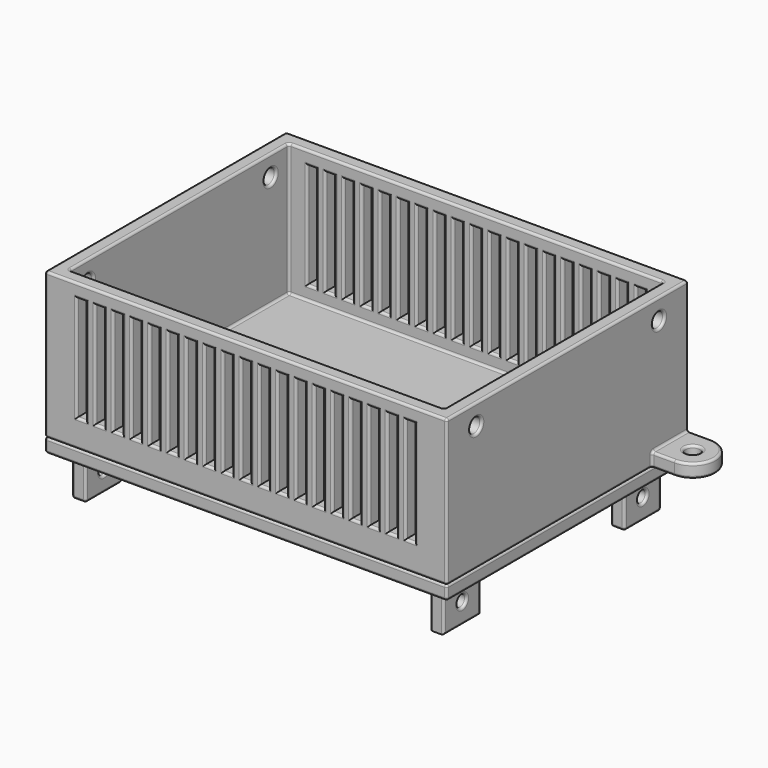
from build123d import *

# Parameters (mm, degrees)
F5_W           = 82
F5_H           = 60
F6_DEPTH       = 32
F5_W_2         = 3
F5_H_2         = 10
F5_W_3         = 2
F5_H_3         = 3
F5_R           = 3.5
F5_R_2         = 1.6
F7_DEPTH       = 3
F8_DEPTH       = 3
F9_DEPTH       = 1
F10_DEPTH      = 12
F11_DEPTH      = 1
F12_R          = 1.25
F12_R_2        = 1.6
F13_DEPTH      = 85
F13_DEPTH_BACK = 3
F14_W          = 2
F14_H          = 23
F15_DEPTH      = 3
F15_DEPTH_BACK = 63
F16_R          = 0.5
F16_2_R        = 0.5


with BuildPart() as f6:
    # F5 (on Top) → F6 (new body)
    with BuildSketch(Plane.XY):
        Polygon((85, 3), (-3, 3), (-3, -7), (-3, -63), (85, -63), (85, -7), align=None)
        with Locations((41, -30)):
            Rectangle(F5_W, F5_H, mode=Mode.SUBTRACT)
    extrude(amount=F6_DEPTH)

    # F5 (on Top) → F7 (join)
    with BuildSketch(Plane.XY):
        with Locations((41, -30)):
            Rectangle(F5_W, F5_H)
        with Locations((1.8, -54.7)):
            Rectangle(F5_W_2, F5_H_2, mode=Mode.SUBTRACT)
        Polygon((5.4330127019, -46.6423048454), (5, -46.3923048454), (4.5669872981, -46.1423048454), (6.0669872981, -43.5442286341), (6.9330127019, -44.0442286341), align=None, mode=Mode.SUBTRACT)
        with Locations((3, -36)):
            Rectangle(F5_W_3, F5_H_3, mode=Mode.SUBTRACT)
        with Locations((11, -36)):
            Circle(F5_R, mode=Mode.SUBTRACT)
        Polygon((17, -46.3923048454), (16.5669872981, -46.6423048454), (15.0669872981, -44.0442286341), (15.9330127019, -43.5442286341), (17.4330127019, -46.1423048454), align=None, mode=Mode.SUBTRACT)
        Polygon((26.0669872981, -43.5442286341), (26.9330127019, -44.0442286341), (25.4330127019, -46.6423048454), (25, -46.3923048454), (24.5669872981, -46.1423048454), align=None, mode=Mode.SUBTRACT)
        Polygon((35.9330127019, -43.5442286341), (37.4330127019, -46.1423048454), (37, -46.3923048454), (36.5669872981, -46.6423048454), (35.0669872981, -44.0442286341), align=None, mode=Mode.SUBTRACT)
        with Locations((19, -36)):
            Rectangle(F5_W_3, F5_H_3, mode=Mode.SUBTRACT)
        with Locations((23, -36)):
            Rectangle(F5_W_3, F5_H_3, mode=Mode.SUBTRACT)
        with Locations((31, -36)):
            Circle(F5_R, mode=Mode.SUBTRACT)
        with Locations((39, -36)):
            Rectangle(F5_W_3, F5_H_3, mode=Mode.SUBTRACT)
        with Locations((80.2, -54.7)):
            Rectangle(F5_W_2, F5_H_2, mode=Mode.SUBTRACT)
        Polygon((46.0669872981, -43.5442286341), (46.9330127019, -44.0442286341), (45.4330127019, -46.6423048454), (45, -46.3923048454), (44.5669872981, -46.1423048454), align=None, mode=Mode.SUBTRACT)
        Polygon((55.9330127019, -43.5442286341), (57.4330127019, -46.1423048454), (57, -46.3923048454), (56.5669872981, -46.6423048454), (55.0669872981, -44.0442286341), align=None, mode=Mode.SUBTRACT)
        Polygon((66.0669872981, -43.5442286341), (66.9330127019, -44.0442286341), (65.4330127019, -46.6423048454), (65, -46.3923048454), (64.5669872981, -46.1423048454), align=None, mode=Mode.SUBTRACT)
        with Locations((43, -36)):
            Rectangle(F5_W_3, F5_H_3, mode=Mode.SUBTRACT)
        with Locations((51, -36)):
            Circle(F5_R, mode=Mode.SUBTRACT)
        with Locations((59, -36)):
            Rectangle(F5_W_3, F5_H_3, mode=Mode.SUBTRACT)
        with Locations((63, -36)):
            Rectangle(F5_W_3, F5_H_3, mode=Mode.SUBTRACT)
        Polygon((75.9330127019, -43.5442286341), (77.4330127019, -46.1423048454), (77, -46.3923048454), (76.5669872981, -46.6423048454), (75.0669872981, -44.0442286341), align=None, mode=Mode.SUBTRACT)
        with Locations((71, -36)):
            Circle(F5_R, mode=Mode.SUBTRACT)
        with Locations((79, -36)):
            Rectangle(F5_W_3, F5_H_3, mode=Mode.SUBTRACT)
        Polygon((11.5, -27), (11, -27), (10.5, -27), (10.5, -24), (11.5, -24), align=None, mode=Mode.SUBTRACT)
        Polygon((31.5, -24), (31.5, -27), (31, -27), (30.5, -27), (30.5, -24), align=None, mode=Mode.SUBTRACT)
        with Locations((1.8, -5.3)):
            Rectangle(F5_W_2, F5_H_2, mode=Mode.SUBTRACT)
        Polygon((51.5, -24), (51.5, -27), (51, -27), (50.5, -27), (50.5, -24), align=None, mode=Mode.SUBTRACT)
        Polygon((71.5, -24), (71.5, -27), (71, -27), (70.5, -27), (70.5, -24), align=None, mode=Mode.SUBTRACT)
        with Locations((80.2, -5.3)):
            Rectangle(F5_W_2, F5_H_2, mode=Mode.SUBTRACT)
        with Locations((1.8, -5.3)):
            Rectangle(F5_W_2, F5_H_2)
        with Locations((1.8, -54.7)):
            Rectangle(F5_W_2, F5_H_2)
        with Locations((3, -36)):
            Rectangle(F5_W_3, F5_H_3)
        with Locations((11, -36)):
            Circle(F5_R)
        with Locations((19, -36)):
            Rectangle(F5_W_3, F5_H_3)
        with Locations((23, -36)):
            Rectangle(F5_W_3, F5_H_3)
        with Locations((31, -36)):
            Circle(F5_R)
        with Locations((39, -36)):
            Rectangle(F5_W_3, F5_H_3)
        with Locations((43, -36)):
            Rectangle(F5_W_3, F5_H_3)
        with Locations((51, -36)):
            Circle(F5_R)
        with Locations((63, -36)):
            Rectangle(F5_W_3, F5_H_3)
        with Locations((59, -36)):
            Rectangle(F5_W_3, F5_H_3)
        with Locations((71, -36)):
            Circle(F5_R)
        with Locations((79, -36)):
            Rectangle(F5_W_3, F5_H_3)
        with Locations((80.2, -5.3)):
            Rectangle(F5_W_2, F5_H_2)
        with Locations((80.2, -54.7)):
            Rectangle(F5_W_2, F5_H_2)
        Polygon((4.5669872981, -46.1423048454), (5, -46.3923048454), (5.4330127019, -46.6423048454), (6.9330127019, -44.0442286341), (6.0669872981, -43.5442286341), align=None)
        Polygon((15.0669872981, -44.0442286341), (16.5669872981, -46.6423048454), (17, -46.3923048454), (17.4330127019, -46.1423048454), (15.9330127019, -43.5442286341), align=None)
        Polygon((10.5, -27), (11, -27), (11.5, -27), (11.5, -24), (10.5, -24), align=None)
        Polygon((37, -46.3923048454), (37.4330127019, -46.1423048454), (35.9330127019, -43.5442286341), (35.0669872981, -44.0442286341), (36.5669872981, -46.6423048454), align=None)
        Polygon((51, -27), (51.5, -27), (51.5, -24), (50.5, -24), (50.5, -27), align=None)
        Polygon((45.4330127019, -46.6423048454), (46.9330127019, -44.0442286341), (46.0669872981, -43.5442286341), (44.5669872981, -46.1423048454), (45, -46.3923048454), align=None)
        Polygon((57, -46.3923048454), (57.4330127019, -46.1423048454), (55.9330127019, -43.5442286341), (55.0669872981, -44.0442286341), (56.5669872981, -46.6423048454), align=None)
        Polygon((71, -27), (71.5, -27), (71.5, -24), (70.5, -24), (70.5, -27), align=None)
        Polygon((65.4330127019, -46.6423048454), (66.9330127019, -44.0442286341), (66.0669872981, -43.5442286341), (64.5669872981, -46.1423048454), (65, -46.3923048454), align=None)
        Polygon((77, -46.3923048454), (77.4330127019, -46.1423048454), (75.9330127019, -43.5442286341), (75.0669872981, -44.0442286341), (76.5669872981, -46.6423048454), align=None)
        Polygon((31, -27), (31.5, -27), (31.5, -24), (30.5, -24), (30.5, -27), align=None)
        Polygon((25.4330127019, -46.6423048454), (26.9330127019, -44.0442286341), (26.0669872981, -43.5442286341), (24.5669872981, -46.1423048454), (25, -46.3923048454), align=None)
        with BuildLine():
            Line((-3, -7), (-3, 3))
            Line((-3, 3), (-8, 3))
            ThreePointArc((-8, 3), (-13, -2), (-8, -7))
            Line((-8, -7), (-3, -7))
        make_face()
        with Locations((-8, -2)):
            Circle(F5_R_2, mode=Mode.SUBTRACT)
        with BuildLine():
            Line((90, 3), (85, 3))
            Line((85, 3), (85, -7))
            Line((85, -7), (90, -7))
            ThreePointArc((90, -7), (95, -2), (90, 3))
        make_face()
        with Locations((90, -2)):
            Circle(F5_R_2, mode=Mode.SUBTRACT)
    extrude(amount=F7_DEPTH)


with BuildPart() as f8:
    # F5 (on Top) → F8 (new body)
    with BuildSketch(Plane.XY):
        Polygon((85, 3), (-3, 3), (-3, -7), (-3, -63), (85, -63), (85, -7), align=None)
        with Locations((41, -30)):
            Rectangle(F5_W, F5_H, mode=Mode.SUBTRACT)
        with Locations((41, -30)):
            Rectangle(F5_W, F5_H)
        with Locations((1.8, -54.7)):
            Rectangle(F5_W_2, F5_H_2, mode=Mode.SUBTRACT)
        Polygon((5.4330127019, -46.6423048454), (5, -46.3923048454), (4.5669872981, -46.1423048454), (6.0669872981, -43.5442286341), (6.9330127019, -44.0442286341), align=None, mode=Mode.SUBTRACT)
        with Locations((3, -36)):
            Rectangle(F5_W_3, F5_H_3, mode=Mode.SUBTRACT)
        with Locations((11, -36)):
            Circle(F5_R, mode=Mode.SUBTRACT)
        Polygon((17, -46.3923048454), (16.5669872981, -46.6423048454), (15.0669872981, -44.0442286341), (15.9330127019, -43.5442286341), (17.4330127019, -46.1423048454), align=None, mode=Mode.SUBTRACT)
        Polygon((26.0669872981, -43.5442286341), (26.9330127019, -44.0442286341), (25.4330127019, -46.6423048454), (25, -46.3923048454), (24.5669872981, -46.1423048454), align=None, mode=Mode.SUBTRACT)
        Polygon((35.9330127019, -43.5442286341), (37.4330127019, -46.1423048454), (37, -46.3923048454), (36.5669872981, -46.6423048454), (35.0669872981, -44.0442286341), align=None, mode=Mode.SUBTRACT)
        with Locations((19, -36)):
            Rectangle(F5_W_3, F5_H_3, mode=Mode.SUBTRACT)
        with Locations((23, -36)):
            Rectangle(F5_W_3, F5_H_3, mode=Mode.SUBTRACT)
        with Locations((31, -36)):
            Circle(F5_R, mode=Mode.SUBTRACT)
        with Locations((39, -36)):
            Rectangle(F5_W_3, F5_H_3, mode=Mode.SUBTRACT)
        with Locations((80.2, -54.7)):
            Rectangle(F5_W_2, F5_H_2, mode=Mode.SUBTRACT)
        Polygon((46.0669872981, -43.5442286341), (46.9330127019, -44.0442286341), (45.4330127019, -46.6423048454), (45, -46.3923048454), (44.5669872981, -46.1423048454), align=None, mode=Mode.SUBTRACT)
        Polygon((55.9330127019, -43.5442286341), (57.4330127019, -46.1423048454), (57, -46.3923048454), (56.5669872981, -46.6423048454), (55.0669872981, -44.0442286341), align=None, mode=Mode.SUBTRACT)
        Polygon((66.0669872981, -43.5442286341), (66.9330127019, -44.0442286341), (65.4330127019, -46.6423048454), (65, -46.3923048454), (64.5669872981, -46.1423048454), align=None, mode=Mode.SUBTRACT)
        with Locations((43, -36)):
            Rectangle(F5_W_3, F5_H_3, mode=Mode.SUBTRACT)
        with Locations((51, -36)):
            Circle(F5_R, mode=Mode.SUBTRACT)
        with Locations((59, -36)):
            Rectangle(F5_W_3, F5_H_3, mode=Mode.SUBTRACT)
        with Locations((63, -36)):
            Rectangle(F5_W_3, F5_H_3, mode=Mode.SUBTRACT)
        Polygon((75.9330127019, -43.5442286341), (77.4330127019, -46.1423048454), (77, -46.3923048454), (76.5669872981, -46.6423048454), (75.0669872981, -44.0442286341), align=None, mode=Mode.SUBTRACT)
        with Locations((71, -36)):
            Circle(F5_R, mode=Mode.SUBTRACT)
        with Locations((79, -36)):
            Rectangle(F5_W_3, F5_H_3, mode=Mode.SUBTRACT)
        Polygon((11.5, -27), (11, -27), (10.5, -27), (10.5, -24), (11.5, -24), align=None, mode=Mode.SUBTRACT)
        Polygon((31.5, -24), (31.5, -27), (31, -27), (30.5, -27), (30.5, -24), align=None, mode=Mode.SUBTRACT)
        with Locations((1.8, -5.3)):
            Rectangle(F5_W_2, F5_H_2, mode=Mode.SUBTRACT)
        Polygon((51.5, -24), (51.5, -27), (51, -27), (50.5, -27), (50.5, -24), align=None, mode=Mode.SUBTRACT)
        Polygon((71.5, -24), (71.5, -27), (71, -27), (70.5, -27), (70.5, -24), align=None, mode=Mode.SUBTRACT)
        with Locations((80.2, -5.3)):
            Rectangle(F5_W_2, F5_H_2, mode=Mode.SUBTRACT)
        with Locations((1.8, -5.3)):
            Rectangle(F5_W_2, F5_H_2)
        with Locations((1.8, -54.7)):
            Rectangle(F5_W_2, F5_H_2)
        with Locations((80.2, -5.3)):
            Rectangle(F5_W_2, F5_H_2)
        with Locations((80.2, -54.7)):
            Rectangle(F5_W_2, F5_H_2)
        Polygon((10.5, -27), (11, -27), (11.5, -27), (11.5, -24), (10.5, -24), align=None)
        Polygon((4.5669872981, -46.1423048454), (5, -46.3923048454), (5.4330127019, -46.6423048454), (6.9330127019, -44.0442286341), (6.0669872981, -43.5442286341), align=None)
        Polygon((15.0669872981, -44.0442286341), (16.5669872981, -46.6423048454), (17, -46.3923048454), (17.4330127019, -46.1423048454), (15.9330127019, -43.5442286341), align=None)
        Polygon((25.4330127019, -46.6423048454), (26.9330127019, -44.0442286341), (26.0669872981, -43.5442286341), (24.5669872981, -46.1423048454), (25, -46.3923048454), align=None)
        Polygon((37, -46.3923048454), (37.4330127019, -46.1423048454), (35.9330127019, -43.5442286341), (35.0669872981, -44.0442286341), (36.5669872981, -46.6423048454), align=None)
        Polygon((31, -27), (31.5, -27), (31.5, -24), (30.5, -24), (30.5, -27), align=None)
        Polygon((51, -27), (51.5, -27), (51.5, -24), (50.5, -24), (50.5, -27), align=None)
        Polygon((45.4330127019, -46.6423048454), (46.9330127019, -44.0442286341), (46.0669872981, -43.5442286341), (44.5669872981, -46.1423048454), (45, -46.3923048454), align=None)
        Polygon((57, -46.3923048454), (57.4330127019, -46.1423048454), (55.9330127019, -43.5442286341), (55.0669872981, -44.0442286341), (56.5669872981, -46.6423048454), align=None)
        Polygon((65.4330127019, -46.6423048454), (66.9330127019, -44.0442286341), (66.0669872981, -43.5442286341), (64.5669872981, -46.1423048454), (65, -46.3923048454), align=None)
        Polygon((77, -46.3923048454), (77.4330127019, -46.1423048454), (75.9330127019, -43.5442286341), (75.0669872981, -44.0442286341), (76.5669872981, -46.6423048454), align=None)
        Polygon((71, -27), (71.5, -27), (71.5, -24), (70.5, -24), (70.5, -27), align=None)
    extrude(amount=-F8_DEPTH)

    # F5 (on Top) → F9 (join)
    with BuildSketch(Plane.XY):
        with Locations((3, -36)):
            Rectangle(F5_W_3, F5_H_3)
        with Locations((19, -36)):
            Rectangle(F5_W_3, F5_H_3)
        with Locations((23, -36)):
            Rectangle(F5_W_3, F5_H_3)
        with Locations((39, -36)):
            Rectangle(F5_W_3, F5_H_3)
        with Locations((43, -36)):
            Rectangle(F5_W_3, F5_H_3)
        with Locations((59, -36)):
            Rectangle(F5_W_3, F5_H_3)
        with Locations((63, -36)):
            Rectangle(F5_W_3, F5_H_3)
        with Locations((79, -36)):
            Rectangle(F5_W_3, F5_H_3)
    extrude(amount=-F9_DEPTH)

    # F5 (on Top) → F10 (join)
    with BuildSketch(Plane.XY):
        with Locations((1.8, -5.3)):
            Rectangle(F5_W_2, F5_H_2)
        with Locations((1.8, -54.7)):
            Rectangle(F5_W_2, F5_H_2)
        with Locations((80.2, -5.3)):
            Rectangle(F5_W_2, F5_H_2)
        with Locations((80.2, -54.7)):
            Rectangle(F5_W_2, F5_H_2)
    extrude(amount=-F10_DEPTH)

    # F5 (on Top) → F11 (cut)
    with BuildSketch(Plane.XY):
        Polygon((71, -27), (71.5, -27), (71.5, -24), (70.5, -24), (70.5, -27), align=None)
        Polygon((65.4330127019, -46.6423048454), (66.9330127019, -44.0442286341), (66.0669872981, -43.5442286341), (64.5669872981, -46.1423048454), (65, -46.3923048454), align=None)
        Polygon((77, -46.3923048454), (77.4330127019, -46.1423048454), (75.9330127019, -43.5442286341), (75.0669872981, -44.0442286341), (76.5669872981, -46.6423048454), align=None)
        Polygon((57, -46.3923048454), (57.4330127019, -46.1423048454), (55.9330127019, -43.5442286341), (55.0669872981, -44.0442286341), (56.5669872981, -46.6423048454), align=None)
        Polygon((45.4330127019, -46.6423048454), (46.9330127019, -44.0442286341), (46.0669872981, -43.5442286341), (44.5669872981, -46.1423048454), (45, -46.3923048454), align=None)
        Polygon((51, -27), (51.5, -27), (51.5, -24), (50.5, -24), (50.5, -27), align=None)
        Polygon((37, -46.3923048454), (37.4330127019, -46.1423048454), (35.9330127019, -43.5442286341), (35.0669872981, -44.0442286341), (36.5669872981, -46.6423048454), align=None)
        Polygon((25.4330127019, -46.6423048454), (26.9330127019, -44.0442286341), (26.0669872981, -43.5442286341), (24.5669872981, -46.1423048454), (25, -46.3923048454), align=None)
        Polygon((31, -27), (31.5, -27), (31.5, -24), (30.5, -24), (30.5, -27), align=None)
        Polygon((10.5, -27), (11, -27), (11.5, -27), (11.5, -24), (10.5, -24), align=None)
        Polygon((15.0669872981, -44.0442286341), (16.5669872981, -46.6423048454), (17, -46.3923048454), (17.4330127019, -46.1423048454), (15.9330127019, -43.5442286341), align=None)
        Polygon((4.5669872981, -46.1423048454), (5, -46.3923048454), (5.4330127019, -46.6423048454), (6.9330127019, -44.0442286341), (6.0669872981, -43.5442286341), align=None)
    extrude(amount=-F11_DEPTH, mode=Mode.SUBTRACT)


with BuildPart() as f13_tool:
    # F12 (on Right) → F13 (new body, two sides)
    with BuildSketch(Plane.YZ) as f13_sk:
        with Locations((-54.7, -7.5)):
            Circle(F12_R)
        with Locations((-5.3, -7.5)):
            Circle(F12_R)
        with Locations((-5, 27.5)):
            Circle(F12_R_2)
        with Locations((-55, 27.5)):
            Circle(F12_R_2)
    extrude(amount=F13_DEPTH)
    extrude(f13_sk.sketch, amount=-F13_DEPTH_BACK)


with BuildPart() as f6_1:
    add(f6.part)

    # F13: cut by f13_tool
    add(f13_tool.part, mode=Mode.SUBTRACT)

    # F14 (on Front) → F15 (cut, two sides)
    with BuildSketch(Plane.XZ) as f15_sk:
        with Locations((5, 17.5)):
            Rectangle(F14_W, F14_H)
        with Locations((9, 17.5)):
            Rectangle(F14_W, F14_H)
        with Locations((13, 17.5)):
            Rectangle(F14_W, F14_H)
        with Locations((17, 17.5)):
            Rectangle(F14_W, F14_H)
        with Locations((21, 17.5)):
            Rectangle(F14_W, F14_H)
        with Locations((25, 17.5)):
            Rectangle(F14_W, F14_H)
        with Locations((29, 17.5)):
            Rectangle(F14_W, F14_H)
        with Locations((33, 17.5)):
            Rectangle(F14_W, F14_H)
        with Locations((37, 17.5)):
            Rectangle(F14_W, F14_H)
        with Locations((41, 17.5)):
            Rectangle(F14_W, F14_H)
        with Locations((45, 17.5)):
            Rectangle(F14_W, F14_H)
        with Locations((49, 17.5)):
            Rectangle(F14_W, F14_H)
        with Locations((53, 17.5)):
            Rectangle(F14_W, F14_H)
        with Locations((57, 17.5)):
            Rectangle(F14_W, F14_H)
        with Locations((61, 17.5)):
            Rectangle(F14_W, F14_H)
        with Locations((65, 17.5)):
            Rectangle(F14_W, F14_H)
        with Locations((69, 17.5)):
            Rectangle(F14_W, F14_H)
        with Locations((73, 17.5)):
            Rectangle(F14_W, F14_H)
        with Locations((77, 17.5)):
            Rectangle(F14_W, F14_H)
    extrude(amount=-F15_DEPTH, mode=Mode.SUBTRACT)
    extrude(f15_sk.sketch, amount=F15_DEPTH_BACK, mode=Mode.SUBTRACT)

    # F16
    f16_edges = [f6_1.edges().sort_by_distance(p)[0] for p in [
        (-3, -2, 3),
        (-3, -7, 1.5),
        (-3, 3, 17.5),
        (-3, -35, 0),
        (-3, -30, 32),
        (-3, -63, 16),
        (-3, -6.6, 27.5),
        (-3, -56.6, 27.5),
        (85, 3, 17.5),
        (87.5, 3, 3),
        (41, 3, 32),
        (90, 3, 1.5),
        (41, 3, 0),
        (-5.5, 3, 3),
        (-8, 3, 1.5),
        (77, 3, 6),
        (78, 3, 17.5),
        (77, 3, 29),
        (76, 3, 17.5),
        (73, 3, 6),
        (74, 3, 17.5),
        (73, 3, 29),
        (72, 3, 17.5),
        (69, 3, 6),
        (70, 3, 17.5),
        (69, 3, 29),
        (68, 3, 17.5),
        (65, 3, 6),
        (66, 3, 17.5),
        (65, 3, 29),
        (64, 3, 17.5),
        (61, 3, 6),
        (62, 3, 17.5),
        (61, 3, 29),
        (60, 3, 17.5),
        (57, 3, 6),
        (58, 3, 17.5),
        (57, 3, 29),
        (56, 3, 17.5),
        (53, 3, 6),
        (54, 3, 17.5),
        (53, 3, 29),
        (52, 3, 17.5),
        (49, 3, 6),
        (50, 3, 17.5),
        (49, 3, 29),
        (48, 3, 17.5),
        (45, 3, 6),
        (46, 3, 17.5),
        (45, 3, 29),
        (44, 3, 17.5),
        (41, 3, 6),
        (42, 3, 17.5),
        (41, 3, 29),
        (40, 3, 17.5),
        (37, 3, 6),
        (38, 3, 17.5),
        (37, 3, 29),
        (36, 3, 17.5),
        (33, 3, 6),
        (34, 3, 17.5),
        (33, 3, 29),
        (32, 3, 17.5),
        (29, 3, 6),
        (30, 3, 17.5),
        (29, 3, 29),
        (28, 3, 17.5),
        (25, 3, 6),
        (26, 3, 17.5),
        (25, 3, 29),
        (24, 3, 17.5),
        (21, 3, 6),
        (22, 3, 17.5),
        (21, 3, 29),
        (20, 3, 17.5),
        (17, 3, 6),
        (18, 3, 17.5),
        (17, 3, 29),
        (16, 3, 17.5),
        (13, 3, 6),
        (14, 3, 17.5),
        (13, 3, 29),
        (12, 3, 17.5),
        (9, 3, 6),
        (10, 3, 17.5),
        (9, 3, 29),
        (8, 3, 17.5),
        (5, 3, 29),
        (4, 3, 17.5),
        (5, 3, 6),
        (6, 3, 17.5),
        (41, -63, 0),
        (41, -63, 32),
        (85, -63, 16),
        (6, -63, 17.5),
        (5, -63, 6),
        (4, -63, 17.5),
        (5, -63, 29),
        (8, -63, 17.5),
        (9, -63, 29),
        (10, -63, 17.5),
        (9, -63, 6),
        (12, -63, 17.5),
        (13, -63, 29),
        (14, -63, 17.5),
        (13, -63, 6),
        (16, -63, 17.5),
        (17, -63, 29),
        (18, -63, 17.5),
        (17, -63, 6),
        (20, -63, 17.5),
        (21, -63, 29),
        (22, -63, 17.5),
        (21, -63, 6),
        (24, -63, 17.5),
        (25, -63, 29),
        (26, -63, 17.5),
        (25, -63, 6),
        (28, -63, 17.5),
        (29, -63, 29),
        (30, -63, 17.5),
        (29, -63, 6),
        (32, -63, 17.5),
        (33, -63, 29),
        (34, -63, 17.5),
        (33, -63, 6),
        (36, -63, 17.5),
        (37, -63, 29),
        (38, -63, 17.5),
        (37, -63, 6),
        (40, -63, 17.5),
        (41, -63, 29),
        (42, -63, 17.5),
        (41, -63, 6),
        (44, -63, 17.5),
        (45, -63, 29),
        (46, -63, 17.5),
        (45, -63, 6),
        (48, -63, 17.5),
        (49, -63, 29),
        (50, -63, 17.5),
        (49, -63, 6),
        (52, -63, 17.5),
        (53, -63, 29),
        (54, -63, 17.5),
        (53, -63, 6),
        (56, -63, 17.5),
        (57, -63, 29),
        (58, -63, 17.5),
        (57, -63, 6),
        (60, -63, 17.5),
        (61, -63, 29),
        (62, -63, 17.5),
        (61, -63, 6),
        (64, -63, 17.5),
        (65, -63, 29),
        (66, -63, 17.5),
        (65, -63, 6),
        (68, -63, 17.5),
        (69, -63, 29),
        (70, -63, 17.5),
        (69, -63, 6),
        (72, -63, 17.5),
        (73, -63, 29),
        (74, -63, 17.5),
        (73, -63, 6),
        (76, -63, 17.5),
        (77, -63, 29),
        (78, -63, 17.5),
        (77, -63, 6),
        (85, -35, 0),
        (85, -7, 1.5),
        (85, -30, 32),
        (85, -2, 3),
        (85, -56.6, 27.5),
        (85, -6.6, 27.5),
        (-13, -2, 0),
        (-5.5, -7, 0),
        (87.5, -7, 0),
        (95, -2, 0),
        (-9.6, -2, 0),
        (88.4, -2, 0),
        (41, 0, 3),
        (0, -30, 3),
        (41, -60, 3),
        (82, -30, 3),
        (0, 0, 17.5),
        (0, -60, 17.5),
        (0, -30, 32),
        (0, -56.6, 27.5),
        (0, -6.6, 27.5),
        (82, -60, 17.5),
        (82, 0, 17.5),
        (82, -30, 32),
        (82, -6.6, 27.5),
        (82, -56.6, 27.5),
        (41, 0, 32),
        (5, 0, 29),
        (6, 0, 17.5),
        (5, 0, 6),
        (4, 0, 17.5),
        (9, 0, 6),
        (8, 0, 17.5),
        (9, 0, 29),
        (10, 0, 17.5),
        (13, 0, 6),
        (12, 0, 17.5),
        (13, 0, 29),
        (14, 0, 17.5),
        (17, 0, 6),
        (16, 0, 17.5),
        (17, 0, 29),
        (18, 0, 17.5),
        (21, 0, 6),
        (20, 0, 17.5),
        (21, 0, 29),
        (22, 0, 17.5),
        (25, 0, 6),
        (24, 0, 17.5),
        (25, 0, 29),
        (26, 0, 17.5),
        (29, 0, 6),
        (28, 0, 17.5),
        (29, 0, 29),
        (30, 0, 17.5),
        (33, 0, 6),
        (32, 0, 17.5),
        (33, 0, 29),
        (34, 0, 17.5),
        (37, 0, 6),
        (36, 0, 17.5),
        (37, 0, 29),
        (38, 0, 17.5),
        (41, 0, 6),
        (40, 0, 17.5),
        (41, 0, 29),
        (42, 0, 17.5),
        (45, 0, 6),
        (44, 0, 17.5),
        (45, 0, 29),
        (46, 0, 17.5),
        (49, 0, 6),
        (48, 0, 17.5),
        (49, 0, 29),
        (50, 0, 17.5),
        (53, 0, 6),
        (52, 0, 17.5),
        (53, 0, 29),
        (54, 0, 17.5),
        (57, 0, 6),
        (56, 0, 17.5),
        (57, 0, 29),
        (58, 0, 17.5),
        (61, 0, 6),
        (60, 0, 17.5),
        (61, 0, 29),
        (62, 0, 17.5),
        (65, 0, 6),
        (64, 0, 17.5),
        (65, 0, 29),
        (66, 0, 17.5),
        (69, 0, 6),
        (68, 0, 17.5),
        (69, 0, 29),
        (70, 0, 17.5),
        (73, 0, 6),
        (72, 0, 17.5),
        (73, 0, 29),
        (74, 0, 17.5),
        (77, 0, 6),
        (76, 0, 17.5),
        (77, 0, 29),
        (78, 0, 17.5),
        (41, -60, 32),
        (77, -60, 6),
        (78, -60, 17.5),
        (77, -60, 29),
        (76, -60, 17.5),
        (73, -60, 6),
        (74, -60, 17.5),
        (73, -60, 29),
        (72, -60, 17.5),
        (69, -60, 6),
        (70, -60, 17.5),
        (69, -60, 29),
        (68, -60, 17.5),
        (65, -60, 6),
        (66, -60, 17.5),
        (65, -60, 29),
        (64, -60, 17.5),
        (61, -60, 6),
        (62, -60, 17.5),
        (61, -60, 29),
        (60, -60, 17.5),
        (57, -60, 6),
        (58, -60, 17.5),
        (57, -60, 29),
        (56, -60, 17.5),
        (53, -60, 6),
        (54, -60, 17.5),
        (53, -60, 29),
        (52, -60, 17.5),
        (49, -60, 6),
        (50, -60, 17.5),
        (49, -60, 29),
        (48, -60, 17.5),
        (45, -60, 6),
        (46, -60, 17.5),
        (45, -60, 29),
        (44, -60, 17.5),
        (41, -60, 6),
        (42, -60, 17.5),
        (41, -60, 29),
        (40, -60, 17.5),
        (37, -60, 6),
        (38, -60, 17.5),
        (37, -60, 29),
        (36, -60, 17.5),
        (33, -60, 6),
        (34, -60, 17.5),
        (33, -60, 29),
        (32, -60, 17.5),
        (29, -60, 6),
        (30, -60, 17.5),
        (29, -60, 29),
        (28, -60, 17.5),
        (25, -60, 6),
        (26, -60, 17.5),
        (25, -60, 29),
        (24, -60, 17.5),
        (21, -60, 6),
        (22, -60, 17.5),
        (21, -60, 29),
        (20, -60, 17.5),
        (17, -60, 6),
        (18, -60, 17.5),
        (17, -60, 29),
        (16, -60, 17.5),
        (13, -60, 6),
        (14, -60, 17.5),
        (13, -60, 29),
        (12, -60, 17.5),
        (9, -60, 6),
        (10, -60, 17.5),
        (9, -60, 29),
        (8, -60, 17.5),
        (5, -60, 29),
        (4, -60, 17.5),
        (5, -60, 6),
        (6, -60, 17.5),
        (91.6, -2, 1.5),
        (88.4, -2, 3),
        (-6.4, -2, 1.5),
        (-9.6, -2, 3),
        (87.5, -7, 3),
        (95, -2, 3),
        (-5.5, -7, 3),
        (-13, -2, 3),
    ]]
    fillet(f16_edges, radius=F16_R)


with BuildPart() as f8_1:
    add(f8.part)

    # F13: cut by f13_tool
    add(f13_tool.part, mode=Mode.SUBTRACT)

    # F16#2
    f16_2_edges = [f8_1.edges().sort_by_distance(p)[0] for p in [
        (41, 3, 0),
        (41, -63, 0),
        (41, 3, -3),
        (85, -30, -3),
        (-3, -30, -3),
        (41, -63, -3),
        (0.3, -54.7, -3),
        (1.8, -59.7, -3),
        (3.3, -54.7, -3),
        (1.8, -49.7, -3),
        (3, -37.5, -3),
        (4, -36, -3),
        (2, -36, -3),
        (3, -34.5, -3),
        (7.5, -36, -3),
        (18, -36, -3),
        (19, -37.5, -3),
        (19, -34.5, -3),
        (20, -36, -3),
        (23, -37.5, -3),
        (24, -36, -3),
        (22, -36, -3),
        (23, -34.5, -3),
        (27.5, -36, -3),
        (39, -34.5, -3),
        (38, -36, -3),
        (40, -36, -3),
        (39, -37.5, -3),
        (81.7, -54.7, -3),
        (80.2, -49.7, -3),
        (78.7, -54.7, -3),
        (80.2, -59.7, -3),
        (43, -37.5, -3),
        (44, -36, -3),
        (42, -36, -3),
        (43, -34.5, -3),
        (47.5, -36, -3),
        (59, -34.5, -3),
        (58, -36, -3),
        (60, -36, -3),
        (59, -37.5, -3),
        (63, -37.5, -3),
        (64, -36, -3),
        (62, -36, -3),
        (63, -34.5, -3),
        (67.5, -36, -3),
        (79, -34.5, -3),
        (78, -36, -3),
        (80, -36, -3),
        (79, -37.5, -3),
        (0.3, -5.3, -3),
        (1.8, -10.3, -3),
        (3.3, -5.3, -3),
        (1.8, -0.3, -3),
        (80.2, -0.3, -3),
        (78.7, -5.3, -3),
        (80.2, -10.3, -3),
        (81.7, -5.3, -3),
        (85, -30, 0),
        (-3, -30, 0),
        (5.316987, -44.843267, 0),
        (5, -46.392305, 0),
        (6.183013, -45.343267, 0),
        (6.5, -43.794229, 0),
        (15.5, -43.794229, 0),
        (15.816987, -45.343267, 0),
        (17, -46.392305, 0),
        (16.683013, -44.843267, 0),
        (26.183013, -45.343267, 0),
        (26.5, -43.794229, 0),
        (25.316987, -44.843267, 0),
        (25, -46.392305, 0),
        (36.683013, -44.843267, 0),
        (35.5, -43.794229, 0),
        (35.816987, -45.343267, 0),
        (37, -46.392305, 0),
        (7.5, -36, 0),
        (27.5, -36, 0),
        (46.183013, -45.343267, 0),
        (46.5, -43.794229, 0),
        (45.316987, -44.843267, 0),
        (45, -46.392305, 0),
        (56.683013, -44.843267, 0),
        (55.5, -43.794229, 0),
        (55.816987, -45.343267, 0),
        (57, -46.392305, 0),
        (65, -46.392305, 0),
        (66.183013, -45.343267, 0),
        (66.5, -43.794229, 0),
        (65.316987, -44.843267, 0),
        (77, -46.392305, 0),
        (76.683013, -44.843267, 0),
        (75.5, -43.794229, 0),
        (75.816987, -45.343267, 0),
        (47.5, -36, 0),
        (67.5, -36, 0),
        (11, -27, 0),
        (11.5, -25.5, 0),
        (11, -24, 0),
        (10.5, -25.5, 0),
        (31.5, -25.5, 0),
        (31, -24, 0),
        (30.5, -25.5, 0),
        (31, -27, 0),
        (51.5, -25.5, 0),
        (51, -24, 0),
        (50.5, -25.5, 0),
        (51, -27, 0),
        (71.5, -25.5, 0),
        (71, -24, 0),
        (70.5, -25.5, 0),
        (71, -27, 0),
        (81.7, -59.7, -7.5),
        (81.7, -49.7, -7.5),
        (81.7, -54.7, -12),
        (81.7, -55.95, -7.5),
        (81.7, -10.3, -7.5),
        (81.7, -0.3, -7.5),
        (81.7, -5.3, -12),
        (81.7, -6.55, -7.5),
        (3.3, -10.3, -7.5),
        (3.3, -0.3, -7.5),
        (3.3, -5.3, -12),
        (3.3, -6.55, -7.5),
        (3.3, -59.7, -7.5),
        (3.3, -49.7, -7.5),
        (3.3, -54.7, -12),
        (3.3, -55.95, -7.5),
        (0.3, -49.7, -7.5),
        (0.3, -59.7, -7.5),
        (0.3, -54.7, -12),
        (0.3, -55.95, -7.5),
        (0.3, -0.3, -7.5),
        (0.3, -10.3, -7.5),
        (0.3, -5.3, -12),
        (0.3, -6.55, -7.5),
        (78.7, -49.7, -7.5),
        (78.7, -59.7, -7.5),
        (78.7, -54.7, -12),
        (78.7, -55.95, -7.5),
        (78.7, -0.3, -7.5),
        (78.7, -10.3, -7.5),
        (78.7, -5.3, -12),
        (78.7, -6.55, -7.5),
        (1.8, -59.7, -12),
        (1.8, -49.7, -12),
        (1.8, -10.3, -12),
        (1.8, -0.3, -12),
        (80.2, -0.3, -12),
        (80.2, -10.3, -12),
        (85, 3, -1.5),
        (-3, 3, -1.5),
        (-3, -63, -1.5),
        (85, -63, -1.5),
    ]]
    fillet(f16_2_edges, radius=F16_2_R)


solid = Compound([f6_1.part, f8_1.part])
